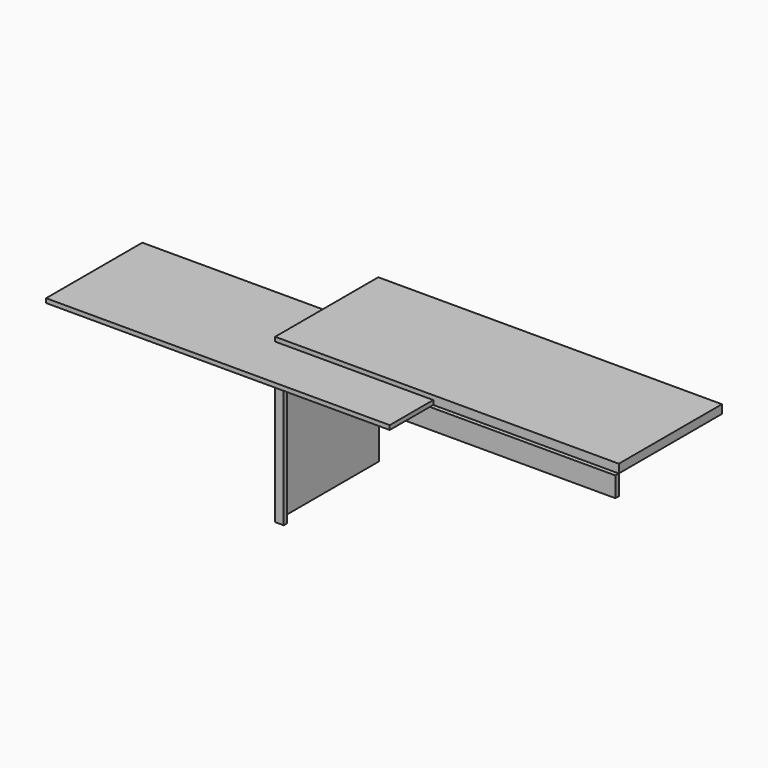
from build123d import *

# Parameters (mm, degrees)
F0_W      = 1524
F0_H      = 571.5
F1_DEPTH  = 38.1
F2_W      = 38.1
F2_H      = 685.8
F3_DEPTH  = 19.05
F4_W      = 533.4
F4_H      = 38.1
F6_DEPTH  = 19.05
F5_W      = 304.8
F5_H      = 38.1
F7_DEPTH  = 19.05
F8_W      = 533.4
F8_H      = 666.75
F9_DEPTH  = 19.05
F10_W     = 1524
F10_H     = 533.4
F11_DEPTH = 19.05
F12_W     = 1524
F12_H     = 88.9
F13_DEPTH = 19.05
F14_W     = 438.15
F14_H     = 88.9
F15_DEPTH = 19.05


# Not quite as in the source:
# - a feature names something its author has since deleted; it is built from what else it names


with BuildPart() as f1:
    # F0 (on Top) → F1 (new body)
    with BuildSketch(Plane.XY):
        with Locations((762, 285.75)):
            Rectangle(F0_W, F0_H)
    extrude(amount=F1_DEPTH)


with BuildPart() as f3:
    # F2 (on Front) → F3 (new body)
    with BuildSketch(Plane.XZ):
        with Locations((19.05, -342.9)):
            Rectangle(F2_W, F2_H)
    extrude(amount=-F3_DEPTH)


with BuildPart() as f6:
    # F4 (on Front) → F6 (new body)
    with BuildSketch(Plane.XZ):
        with Locations((304.8, -19.05)):
            Rectangle(F4_W, F4_H)
    extrude(amount=-F6_DEPTH)


with BuildPart() as f7:
    # F5 (on Front) → F7 (new body)
    with BuildSketch(Plane.XZ):
        with Locations((762, -19.05)):
            Rectangle(F5_W, F5_H)
    extrude(amount=-F7_DEPTH)


with BuildPart() as f9:
    # F8 (on Right) → F9 (new body)
    with BuildSketch(Plane.YZ):
        with Locations((285.75, -333.375)):
            Rectangle(F8_W, F8_H)
    extrude(amount=F9_DEPTH)


with BuildPart() as f11:
    # F10 (on Top) → F11 (new body)
    with BuildSketch(Plane.XY):
        with Locations((-60.9013997018, 25.5651345968)):
            Rectangle(F10_W, F10_H)
    extrude(amount=F11_DEPTH)


with BuildPart() as f13:
    # F12 (on Front) → F13 (new body)
    with BuildSketch(Plane.XZ):
        with Locations((762, -44.45)):
            Rectangle(F12_W, F12_H)
    extrude(amount=F13_DEPTH)


with BuildPart() as f15:
    # F14 (on Right) → F15 (new body)
    with BuildSketch(Plane.YZ):
        with Locations((263.525, -46.7950011114)):
            Rectangle(F14_W, F14_H)
    extrude(amount=F15_DEPTH)


solid = Compound([f1.part, f3.part, f6.part, f7.part, f9.part, f11.part, f13.part, f15.part])
